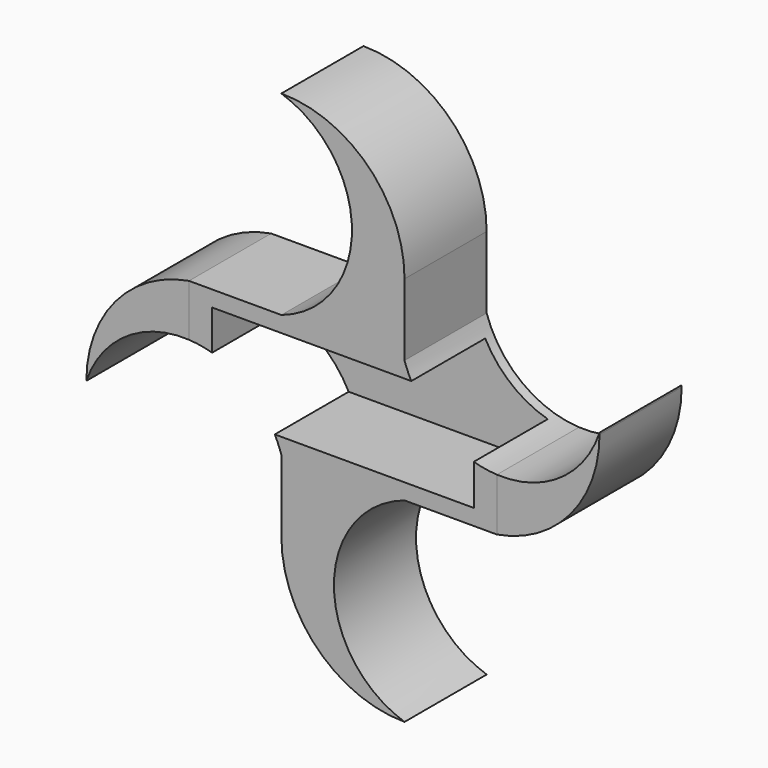
from build123d import *

# Parameters (mm, degrees)
F0_W           = 25.5
F0_H           = 8.9
F1_DEPTH       = 8.9
F2_W           = 30
F2_H           = 12
F2_W_2         = 25.5
F2_H_2         = 8.9
F3_DEPTH       = 10
F4_DEPTH       = 9
F5_DEPTH       = 10
F6_DEPTH       = 10
F8_DEPTH       = 19
F10_DEPTH      = 19
F11_F1_R       = 11.9999
F11_F2_R       = 11.9999
F11_2_T1_DEPTH = 69.160797831
F11_3_T1_DEPTH = 69.160797831
F13_DEPTH      = 10


# Not quite as in the source:
# - a fillet or chamfer that OpenCascade refuses, or shapes differently, is made with other operations: its cross-section is extruded or revolved along the edge and cut away or added
# - a fillet or chamfer is up to 0.001 mm smaller than in the source, because OpenCascade refuses the exact size


with BuildPart() as f1:
    # F0 (on Top) → F1 (new body)
    with BuildSketch(Plane.XY):
        with Locations((12.75, 4.45)):
            Rectangle(F0_W, F0_H)
    extrude(amount=F1_DEPTH)


with BuildPart() as f3:
    # F2 (on face) → F3 (new body)
    with BuildSketch(Plane.XZ):
        with Locations((12.75, 4.45)):
            Rectangle(F2_W, F2_H)
        with Locations((12.75, 4.45)):
            Rectangle(F2_W_2, F2_H_2, mode=Mode.SUBTRACT)
        with Locations((12.75, 4.45)):
            Rectangle(F2_W_2, F2_H_2)
    extrude(amount=-F3_DEPTH)


with BuildPart() as f4_tool:
    # F4 (cut): a face of the model
    f4_faces = [f1.part.faces().sort_by_distance(p)[0] for p in [
        (12.75, 0, 4.45),
    ]]
    extrude(f4_faces, amount=-F4_DEPTH)


with BuildPart() as f1_1:
    add(f1.part)

    # F4: cut by f4_tool
    add(f4_tool.part, mode=Mode.SUBTRACT)


with BuildPart() as f3_1:
    add(f3.part)

    # F4: cut by f4_tool
    add(f4_tool.part, mode=Mode.SUBTRACT)


with BuildPart() as f5:
    # F5 (new): a face of the model
    f5_faces = [f3_1.part.faces().sort_by_distance(p)[0] for p in [
        (-2.25, 5, 4.45),
    ]]
    extrude(f5_faces, amount=F5_DEPTH)

    # F11#2: fillet of radius 12 on 1 edges, made by hand

    # F11_2_s2 → F11_2_t1 (cut)
    with BuildSketch(Plane.XZ.offset(-39.5803989155)):
        with BuildLine():
            ThreePointArc((-2.25, 10.45), (-9.4151513899, 6.3638071262), (-12.25, -1.3821595662))
            Line((-12.25, -1.3821595662), (-12.25, 10.45))
            Line((-12.25, 10.45), (-2.25, 10.45))
        make_face()
    extrude(amount=F11_2_T1_DEPTH, mode=Mode.SUBTRACT)


with BuildPart() as f6:
    # F6 (new): a face of the model
    f6_faces = [f3_1.part.faces().sort_by_distance(p)[0] for p in [
        (27.75, 5, 4.45),
    ]]
    extrude(f6_faces, amount=F6_DEPTH)

    # F11#3: fillet of radius 12 on 1 edges, made by hand

    # F11_3_s2 → F11_3_t1 (cut)
    with BuildSketch(Plane.XZ.offset(-39.5803989155)):
        with BuildLine():
            ThreePointArc((27.75, -1.55), (34.9151513899, 2.5361928738), (37.75, 10.2821595662))
            Line((37.75, 10.2821595662), (37.75, -1.55))
            Line((37.75, -1.55), (27.75, -1.55))
        make_face()
    extrude(amount=F11_3_T1_DEPTH, mode=Mode.SUBTRACT)


with BuildPart() as f3_2:
    add(f3_1.part)

    # F7 (on face) → F8 (join)
    with BuildSketch(Plane.XY.offset(10.45)):
        Polygon((6.75, 0), (12.75, 0), (18.75, 0), (18.75, 10), (12.75, 10), (6.75, 10), align=None)
    extrude(amount=F8_DEPTH)

    # F9 (on face) → F10 (join)
    with BuildSketch(Plane(origin=(0, 0, -1.55), x_dir=(1, 0, 0), z_dir=(0, 0, -1))):
        Polygon((6.75, -10), (12.75, -10), (18.75, -10), (18.75, 0), (12.75, 0), (6.75, 0), align=None)
    extrude(amount=F10_DEPTH)

    # F11: fillet of radius 12 on 2 edges, made by hand

    # F11_f1 (radius 12 in the source; OpenCascade refuses exactly that, so slightly less here)
    f11_f1_edges = [f3_2.edges().sort_by_distance(p)[0] for p in [
        (18.75, 5, 29.45),
    ]]
    fillet(f11_f1_edges, radius=F11_F1_R)

    # F11_f2 (radius 12 in the source; OpenCascade refuses exactly that, so slightly less here)
    f11_f2_edges = [f3_2.edges().sort_by_distance(p)[0] for p in [
        (6.75, 5, -20.55),
    ]]
    fillet(f11_f2_edges, radius=F11_F2_R)


with BuildPart() as f13_tool:
    # F12 (on face) → F13 (new body)
    with BuildSketch(Plane(origin=(0, 10, 0), x_dir=(-1, 0, 0), z_dir=(0, 1, 0))):
        with BuildLine():
            Line((-27.75, 3.5850068215), (-27.75, 10.45))
            Line((-27.75, 10.45), (-37.75, 10.45))
            ThreePointArc((-37.75, 10.45), (-33.9096848707, 5.3282302527), (-27.75, 3.5850068215))
        make_face()
        with BuildLine():
            ThreePointArc((-27.75, 3.5850068215), (-22.1851807253, 5.6215262811), (-18.75, 10.45))
            Line((-18.75, 10.45), (-27.75, 10.45))
            Line((-27.75, 10.45), (-27.75, 3.5850068215))
        make_face()
        with BuildLine():
            ThreePointArc((-6.75, 29.45), (-13.6275010008, 19.95), (-6.75, 10.45))
            Line((-6.75, 10.45), (-6.75, 29.45))
        make_face()
        with BuildLine():
            Line((2.25, 5.3987446019), (2.25, -1.55))
            Line((2.25, -1.55), (12.25, -1.55))
            Line((12.25, -1.55), (12.25, -1.3821595662))
            ThreePointArc((12.25, -1.3821595662), (8.389860126, 3.6892779702), (2.25, 5.3987446019))
        make_face()
        with BuildLine():
            ThreePointArc((2.25, 5.3987446019), (-3.3337079529, 3.3279886569), (-6.75, -1.55))
            Line((-6.75, -1.55), (2.25, -1.55))
            Line((2.25, -1.55), (2.25, 5.3987446019))
        make_face()
        with BuildLine():
            ThreePointArc((-18.75, -20.55), (-11.8724989992, -11.05), (-18.75, -1.55))
            Line((-18.75, -1.55), (-18.75, -20.55))
        make_face()
    extrude(amount=-F13_DEPTH)


with BuildPart() as f3_3:
    add(f3_2.part)

    # F13: cut by f13_tool
    add(f13_tool.part, mode=Mode.SUBTRACT)


with BuildPart() as f5_1:
    add(f5.part)

    # F13: cut by f13_tool
    add(f13_tool.part, mode=Mode.SUBTRACT)


with BuildPart() as f6_1:
    add(f6.part)

    # F13: cut by f13_tool
    add(f13_tool.part, mode=Mode.SUBTRACT)


solid = Compound([f3_3.part, f5_1.part, f6_1.part])
